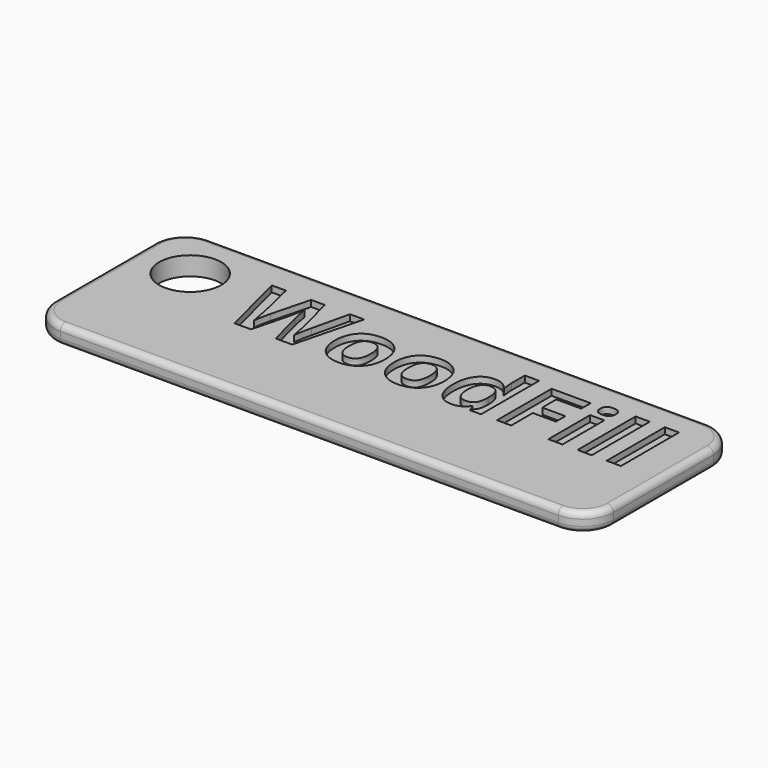
from build123d import *

# Parameters (mm, degrees)
F0_W         = 90
F0_H         = 30
F1_DEPTH     = 3
F2_R         = 1
F3_T1_DEPTH  = 3
F3_T4_ANGLE  = 90
F3_T6_ANGLE  = 90
F3_T8_ANGLE  = 90
F3_T10_ANGLE = 90
F3_T12_ANGLE = 90
F3_T14_ANGLE = 90
F3_T16_ANGLE = 90
F3_T18_ANGLE = 90
F4_R         = 5
F5_DEPTH     = 3
F6_TEXT_SIZE = 15.3874175804
F7_DEPTH     = 1


# Not quite as in the source:
# - a fillet or chamfer that OpenCascade refuses, or shapes differently, is made with other operations: its cross-section is extruded or revolved along the edge and cut away or added
# - Text() gives the source's letters only with a copy of the font that has no kerning and outlines rounded to 1/6400 em; it was checked with that copy


with BuildPart() as f1:
    # F0 (on Top) → F1 (new body)
    with BuildSketch(Plane.XY):
        Rectangle(F0_W, F0_H)
    extrude(amount=F1_DEPTH)

    # F2
    f2_edges = [f1.edges().sort_by_distance(p)[0] for p in [
        (0, 15, 3),
        (-45, 0, 3),
        (0, -15, 3),
        (45, 0, 3),
        (0, 15, 0),
        (-45, 0, 0),
        (0, -15, 0),
        (45, 0, 0),
    ]]
    fillet(f2_edges, radius=F2_R)

    # F3: fillet of radius 5 on 4 edges, made by hand

    # F3_s2 → F3_t1 (cut)
    with BuildSketch(Plane.XY):
        with BuildLine():
            ThreePointArc((45.0004, -9.9990343146), (43.5355339059, -13.5355339059), (39.9990343146, -15.0004))
            Line((39.9990343146, -15.0004), (39.9990343146, -15.5005365685))
            ThreePointArc((39.9990343146, -15.5005365685), (42.4995171573, -15.5001365685), (45, -15.5001365685))
            Line((45, -15.5001365685), (45.5001365685, -15))
            ThreePointArc((45.5001365685, -15), (45.5001365685, -12.4995171573), (45.5005365685, -9.9990343146))
            Line((45.5005365685, -9.9990343146), (45.0004, -9.9990343146))
        make_face()
        with BuildLine():
            ThreePointArc((39.9990343146, 15.0004), (43.5355339059, 13.5355339059), (45.0004, 9.9990343146))
            Line((45.0004, 9.9990343146), (45.5005365685, 9.9990343146))
            ThreePointArc((45.5005365685, 9.9990343146), (45.5001365685, 12.4995171573), (45.5001365685, 15))
            Line((45.5001365685, 15), (45, 15.5001365685))
            ThreePointArc((45, 15.5001365685), (42.4995171573, 15.5001365685), (39.9990343146, 15.5005365685))
            Line((39.9990343146, 15.5005365685), (39.9990343146, 15.0004))
        make_face()
        with BuildLine():
            ThreePointArc((-39.9990343146, 15.0004), (-43.5355339059, 13.5355339059), (-45.0004, 9.9990343146))
            Line((-45.0004, 9.9990343146), (-45.5005365685, 9.9990343146))
            ThreePointArc((-45.5005365685, 9.9990343146), (-45.5001365685, 12.4995171573), (-45.5001365685, 15))
            Line((-45.5001365685, 15), (-45, 15.5001365685))
            ThreePointArc((-45, 15.5001365685), (-42.4995171573, 15.5001365685), (-39.9990343146, 15.5005365685))
            Line((-39.9990343146, 15.5005365685), (-39.9990343146, 15.0004))
        make_face()
        with BuildLine():
            ThreePointArc((-45.0004, -9.9990343146), (-43.5355339059, -13.5355339059), (-39.9990343146, -15.0004))
            Line((-39.9990343146, -15.0004), (-39.9990343146, -15.5005365685))
            ThreePointArc((-39.9990343146, -15.5005365685), (-42.4995171573, -15.5001365685), (-45, -15.5001365685))
            Line((-45, -15.5001365685), (-45.5001365685, -15))
            ThreePointArc((-45.5001365685, -15), (-45.5001365685, -12.4995171573), (-45.5005365685, -9.9990343146))
            Line((-45.5005365685, -9.9990343146), (-45.0004, -9.9990343146))
        make_face()
    extrude(amount=F3_T1_DEPTH, mode=Mode.SUBTRACT)

    # F3_s3 → F3_t4 (revolve, cut)
    with BuildSketch(Plane.YZ.offset(-39.9990343146)):
        with BuildLine():
            ThreePointArc((-14.0004, 0), (-14.7075067812, 0.2928932188), (-15.0004, 1))
            Line((-15.0004, 1), (-15.0004, 0))
            Line((-15.0004, 0), (-14.0004, 0))
        make_face()
    revolve(axis=Axis((-39.9990343146, -9.9990343146, 0), (0, 0, -1)), revolution_arc=F3_T4_ANGLE, mode=Mode.SUBTRACT)

    # F3_s5 → F3_t6 (revolve, cut)
    with BuildSketch(Plane.XZ.offset(9.9990343146)):
        with BuildLine():
            ThreePointArc((-44.0004, 3), (-44.7075067812, 2.7071067812), (-45.0004, 2))
            Line((-45.0004, 2), (-45.0004, 3))
            Line((-45.0004, 3), (-44.0004, 3))
        make_face()
    revolve(axis=Axis((-39.9990343146, -9.9990343146, 3), (0, 0, 1)), revolution_arc=F3_T6_ANGLE, mode=Mode.SUBTRACT)

    # F3_s7 → F3_t8 (revolve, cut)
    with BuildSketch(Plane.XZ.offset(-9.9990343146)):
        with BuildLine():
            ThreePointArc((-44.0004, 0), (-44.7075067812, 0.2928932188), (-45.0004, 1))
            Line((-45.0004, 1), (-45.0004, 0))
            Line((-45.0004, 0), (-44.0004, 0))
        make_face()
    revolve(axis=Axis((-39.9990343146, 9.9990343146, 0), (0, 0, -1)), revolution_arc=F3_T8_ANGLE, mode=Mode.SUBTRACT)

    # F3_s9 → F3_t10 (revolve, cut)
    with BuildSketch(Plane.YZ.offset(-39.9990343146)):
        with BuildLine():
            ThreePointArc((14.0004, 3), (14.7075067812, 2.7071067812), (15.0004, 2))
            Line((15.0004, 2), (15.0004, 3))
            Line((15.0004, 3), (14.0004, 3))
        make_face()
    revolve(axis=Axis((-39.9990343146, 9.9990343146, 3), (0, 0, 1)), revolution_arc=F3_T10_ANGLE, mode=Mode.SUBTRACT)

    # F3_s11 → F3_t12 (revolve, cut)
    with BuildSketch(Plane.YZ.offset(39.9990343146)):
        with BuildLine():
            ThreePointArc((14.0004, 0), (14.7075067812, 0.2928932188), (15.0004, 1))
            Line((15.0004, 1), (15.0004, 0))
            Line((15.0004, 0), (14.0004, 0))
        make_face()
    revolve(axis=Axis((39.9990343146, 9.9990343146, 0), (0, 0, -1)), revolution_arc=F3_T12_ANGLE, mode=Mode.SUBTRACT)

    # F3_s13 → F3_t14 (revolve, cut)
    with BuildSketch(Plane.XZ.offset(-9.9990343146)):
        with BuildLine():
            ThreePointArc((44.0004, 3), (44.7075067812, 2.7071067812), (45.0004, 2))
            Line((45.0004, 2), (45.0004, 3))
            Line((45.0004, 3), (44.0004, 3))
        make_face()
    revolve(axis=Axis((39.9990343146, 9.9990343146, 3), (0, 0, 1)), revolution_arc=F3_T14_ANGLE, mode=Mode.SUBTRACT)

    # F3_s15 → F3_t16 (revolve, cut)
    with BuildSketch(Plane.XZ.offset(9.9990343146)):
        with BuildLine():
            ThreePointArc((44.0004, 0), (44.7075067812, 0.2928932188), (45.0004, 1))
            Line((45.0004, 1), (45.0004, 0))
            Line((45.0004, 0), (44.0004, 0))
        make_face()
    revolve(axis=Axis((39.9990343146, -9.9990343146, 0), (0, 0, -1)), revolution_arc=F3_T16_ANGLE, mode=Mode.SUBTRACT)

    # F3_s17 → F3_t18 (revolve, cut)
    with BuildSketch(Plane.YZ.offset(39.9990343146)):
        with BuildLine():
            ThreePointArc((-14.0004, 3), (-14.7075067812, 2.7071067812), (-15.0004, 2))
            Line((-15.0004, 2), (-15.0004, 3))
            Line((-15.0004, 3), (-14.0004, 3))
        make_face()
    revolve(axis=Axis((39.9990343146, -9.9990343146, 3), (0, 0, 1)), revolution_arc=F3_T18_ANGLE, mode=Mode.SUBTRACT)

    # F4 (on face) → F5 (cut)
    with BuildSketch(Plane.XY.offset(3)):
        with Locations((-36, 6)):
            Circle(F4_R)
    extrude(amount=-F5_DEPTH, mode=Mode.SUBTRACT)

    # F6 (on face) → F7 (cut)
    with BuildSketch(Plane.XY.offset(3)):
        with Locations((-26, -1.0789406579)):
            Text('WoodFill', F6_TEXT_SIZE, font='Open Sans', font_style=FontStyle.BOLD, text_align=(TextAlign.LEFT, TextAlign.BOTTOM))
    extrude(amount=-F7_DEPTH, mode=Mode.SUBTRACT)


solid = f1.part
